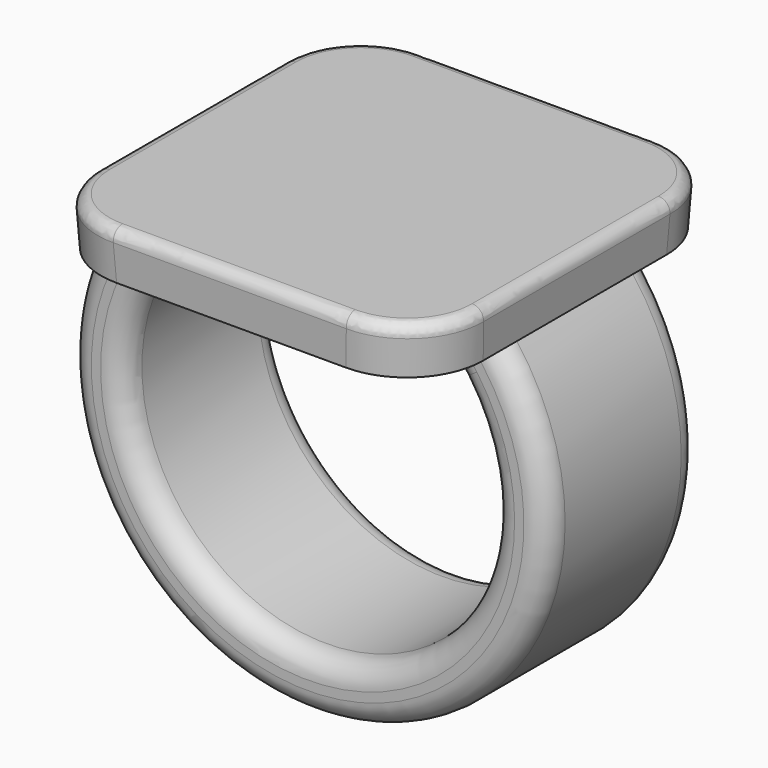
from build123d import *

# Parameters (mm, degrees)
F0_W          = 25.4
F0_H          = 25.4
F1_DEPTH      = 3.175
F1_TAPER      = -3
F3_W          = 5.08
F3_H          = 12.7
F6_DEPTH      = 6.35
F6_DEPTH_BACK = 6.35
F7_R          = 5.08
F8_R          = 1.524
F9_R          = 0.762


with BuildPart() as f1:
    # F0 (on Top) → F1 (new body)
    with BuildSketch(Plane.XY):
        Rectangle(F0_W, F0_H)
    extrude(amount=F1_DEPTH, taper=F1_TAPER)

    # F4: sweep along a path in F2
    with BuildLine(Plane.XZ) as f4_path:
        ThreePointArc((-10.16, 0), (0, -23.5582897328), (10.16, 0))
    # F3 (on face) → F4 (sweep)
    with BuildSketch(Plane(origin=(0, 0, 0), x_dir=(1, 0, 0), z_dir=(0, 0, -1))):
        with Locations((-10.16, 0)):
            Rectangle(F3_W, F3_H)
    sweep(path=f4_path.line)

    # F5 (on Front) → F6 (join, two sides)
    with BuildSketch(Plane.XZ) as f6_sk:
        with BuildLine():
            ThreePointArc((7.62, 0), (8.9072265211, -1.1822790439), (10.0130578512, -2.535746045))
            Line((10.0130578512, -2.535746045), (10.16, 0))
            Line((10.16, 0), (7.62, 0))
        make_face()
    extrude(amount=F6_DEPTH)
    extrude(f6_sk.sketch, amount=-F6_DEPTH_BACK)

    # F7
    f7_edges = [f1.edges().sort_by_distance(p)[0] for p in [
        (12.783197, -12.783197, 1.5875),
        (12.783197, 12.783197, 1.5875),
        (-12.783197, 12.783197, 1.5875),
        (-12.783197, -12.783197, 1.5875),
    ]]
    fillet(f7_edges, radius=F7_R)

    # F8
    f8_edges = [f1.edges().sort_by_distance(p)[0] for p in [
        (-1.743325, 6.35, -21.711017),
        (-1.743325, -6.35, -21.711017),
        (8.907227, -6.35, -1.182279),
        (0, 6.35, -25.501344),
        (0, -6.35, -25.501344),
        (8.907227, 6.35, -1.182279),
    ]]
    fillet(f8_edges, radius=F8_R)

    # F9
    f9_edges = [f1.edges().sort_by_distance(p)[0] for p in [
        (12.866395, 0, 3.175),
        (11.381378, -11.381378, 3.175),
        (11.381378, 11.381378, 3.175),
        (0, -12.866395, 3.175),
        (0, 12.866395, 3.175),
        (-11.381378, -11.381378, 3.175),
        (-11.381378, 11.381378, 3.175),
        (-12.866395, 0, 3.175),
    ]]
    fillet(f9_edges, radius=F9_R)


solid = f1.part
